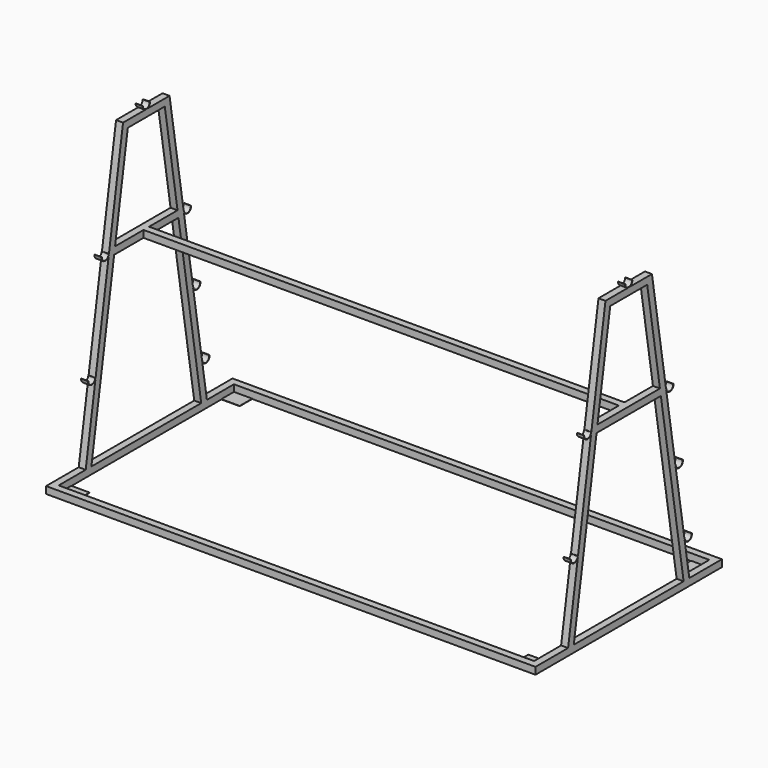
from build123d import *

# Parameters (mm, degrees)
F2_DEPTH  = 38.1
F5_DEPTH  = 38.1
F7_W      = 38.1000000541
F7_H      = 38.1
F8_DEPTH  = 2590.8
F10_DEPTH = 2628.9
F12_W     = 100.0124999999
F12_H     = 85.725
F13_DEPTH = 1.524


# Not quite as in the source:
# - an extrude ends at something that could not be found from the text; its depth is read off the source's solid
# - ends of sketch curves that miss each other by under 0.0002 mm in the source are joined


with BuildPart() as f2:
    # F1 (on Right) → F2 (new body)
    with BuildSketch(Plane.YZ):
        Polygon((634.9999999459, 0.0117264176), (412.7499999459, 0.0117264176), (158.2933200412, 1562.1117264176), (0, 1562.1117264176), (-158.2933200412, 1562.1117264176), (-412.7499999459, 0.0117264176), (-634.9999999459, 0.0117264176), (-634.9999999459, -38.0882735824), (5.41e-08, -38.0882735824), (634.9999999459, -38.0882735824), align=None)
        Polygon((218.9908951289, 952.644992336), (374.1500007125, 0.0247576549), (0, 0.0247576549), (-374.1500007125, 0.0247576549), (-218.9908951289, 952.644992336), (0, 952.644992336), align=None, mode=Mode.SUBTRACT)
        Polygon((125.9288876334, 1524.0117264176), (212.785315444, 990.7449849442), (0, 990.7449849442), (-212.785315444, 990.7449849442), (-125.9288876334, 1524.0117264176), (0, 1524.0052894621), align=None, mode=Mode.SUBTRACT)
    extrude(amount=F2_DEPTH)


with BuildPart() as f3_1:
    # F3: instance of F2
    add(f2.part.mirror(Plane.YZ.offset(-1295.4)))


with BuildPart() as f5:
    # F4 (on Right) → F5 (new body)
    with BuildSketch(Plane.YZ):
        with BuildLine():
            Line((256.5800290113, 971.8518066202), (254.554561688, 971.6889996104))
            ThreePointArc((254.554561688, 971.6889996104), (281.9079908515, 948.4057456927), (305.1912447692, 975.7591748562))
            Line((305.1912447692, 975.7591748562), (303.165777446, 975.5963678464))
            ThreePointArc((303.165777446, 975.5963678464), (281.7451838417, 950.4312130159), (256.5800290113, 971.8518066202))
        make_face()
    extrude(amount=F5_DEPTH)


with BuildPart() as f5b:
    # F4 (on Right) → F5, piece 2 (new body)
    with BuildSketch(Plane.YZ):
        with BuildLine():
            Line((430.2698480282, 208.4277475534), (428.2642817252, 208.1010553365))
            ThreePointArc((428.2642817252, 208.1010553365), (408.9572297354, 181.280082359), (382.1362567578, 200.5871343488))
            Line((382.1362567578, 200.5871343488), (380.1306904549, 200.260442132))
            ThreePointArc((380.1306904549, 200.260442132), (409.2839219522, 179.2745160561), (430.2698480282, 208.4277475534))
        make_face()
    extrude(amount=F5_DEPTH)


with BuildPart() as f5c:
    # F4 (on Right) → F5, piece 3 (new body)
    with BuildSketch(Plane.YZ):
        with BuildLine():
            Line((320.6340097877, 578.1471183433), (318.6284438739, 577.8204237375))
            ThreePointArc((318.6284438739, 577.8204237375), (347.7817003689, 556.8345323879), (368.7675917185, 585.987788883))
            Line((368.7675917185, 585.987788883), (366.7620258047, 585.6610942772))
            ThreePointArc((366.7620258047, 585.6610942772), (347.4550057631, 558.8400983017), (320.6340097877, 578.1471183433))
        make_face()
    extrude(amount=F5_DEPTH)


with BuildPart() as f5d:
    # F4 (on Right) → F5, piece 4 (new body)
    with BuildSketch(Plane.YZ):
        with BuildLine():
            ThreePointArc((-305.1912447692, 975.7591748562), (-281.9079908515, 948.4057456927), (-254.554561688, 971.6889996104))
            Line((-254.554561688, 971.6889996104), (-256.5800290113, 971.8518066202))
            ThreePointArc((-256.5800290113, 971.8518066202), (-281.7451838417, 950.4312130159), (-303.165777446, 975.5963678464))
            Line((-303.165777446, 975.5963678464), (-305.1912447692, 975.7591748562))
        make_face()
    extrude(amount=F5_DEPTH)


with BuildPart() as f5e:
    # F4 (on Right) → F5, piece 5 (new body)
    with BuildSketch(Plane.YZ):
        with BuildLine():
            ThreePointArc((-396.0543227014, 417.9541524412), (-372.7710687837, 390.6007232777), (-345.4176396202, 413.8839771954))
            Line((-345.4176396202, 413.8839771954), (-347.4431069434, 414.0467842053))
            ThreePointArc((-347.4431069434, 414.0467842053), (-372.6082617739, 392.626190601), (-394.0288553782, 417.7913454314))
            Line((-394.0288553782, 417.7913454314), (-396.0543227014, 417.9541524412))
        make_face()
    extrude(amount=F5_DEPTH)


with BuildPart() as f5f:
    # F4 (on Right) → F5, piece 6 (new body)
    with BuildSketch(Plane.YZ):
        with BuildLine():
            Line((-23.368, 1587.5117264176), (-25.4, 1587.5117264176))
            ThreePointArc((-25.4, 1587.5117264176), (0, 1562.1117264176), (25.4, 1587.5117264176))
            Line((25.4, 1587.5117264176), (23.368, 1587.5117264176))
            ThreePointArc((23.368, 1587.5117264176), (0, 1564.1437264176), (-23.368, 1587.5117264176))
        make_face()
    extrude(amount=F5_DEPTH)


with BuildPart() as f6_1:
    # F6: instance of F5d
    add(f5d.part.mirror(Plane.YZ.offset(-1295.4)))


with BuildPart() as f6_2:
    # F6: instance of F5e
    add(f5e.part.mirror(Plane.YZ.offset(-1295.4)))


with BuildPart() as f6_3:
    # F6: instance of F5f
    add(f5f.part.mirror(Plane.YZ.offset(-1295.4)))


with BuildPart() as f6_4:
    # F6: instance of F5
    add(f5.part.mirror(Plane.YZ.offset(-1295.4)))


with BuildPart() as f6_5:
    # F6: instance of F5c
    add(f5c.part.mirror(Plane.YZ.offset(-1295.4)))


with BuildPart() as f6_6:
    # F6: instance of F5b
    add(f5b.part.mirror(Plane.YZ.offset(-1295.4)))


with BuildPart() as f2_1:
    add(f2.part)

    add(f3_1.part)  # F8 merges F3_1
    # F7 (on Right) → F8 (join, through all)
    with BuildSketch(Plane.YZ):
        with Locations((615.9499999729, -19.0382735824)):
            Rectangle(F7_W, F7_H)
        with Locations((-615.9499999729, -19.0382735824)):
            Rectangle(F7_W, F7_H)
    extrude(amount=-F8_DEPTH)

    # F9 (on Right) → F10 (join, through all)
    with BuildSketch(Plane.YZ):
        Polygon((19.05, 990.7449849442), (0, 990.7449849442), (-19.05, 990.7449849442), (-19.05, 952.6449849442), (0, 952.6449849442), (19.05, 952.6449849442), align=None)
    extrude(amount=-F10_DEPTH)

    # F12 (on offset) → F13 (join)
    with BuildSketch(Plane(origin=(0, 0, -38.0882735824), x_dir=(1, 0, 0), z_dir=(0, 0, -1))):
        with Locations((-50.0062500002, -554.0374999459)):
            Rectangle(F12_W, F12_H)
        with Locations((-50.0062500001, 554.0374999459)):
            Rectangle(F12_W, F12_H)
    extrude(amount=-F13_DEPTH)



with BuildPart() as f2_2:
    add(f2_1.part)

    add(f5.part)  # F14 merges F5

    add(f5b.part)  # F14 merges F5b

    add(f5c.part)  # F14 merges F5c

    add(f5d.part)  # F14 merges F5d

    add(f5e.part)  # F14 merges F5e

    add(f5f.part)  # F14 merges F5f

    add(f6_1.part)  # F14 merges F6_1

    add(f6_2.part)  # F14 merges F6_2

    add(f6_3.part)  # F14 merges F6_3

    add(f6_4.part)  # F14 merges F6_4

    add(f6_5.part)  # F14 merges F6_5

    add(f6_6.part)  # F14 merges F6_6
    # F14: F2 across plane
    add(f2_1.part.mirror(Plane.YZ.offset(-1295.4)))


solid = f2_2.part
